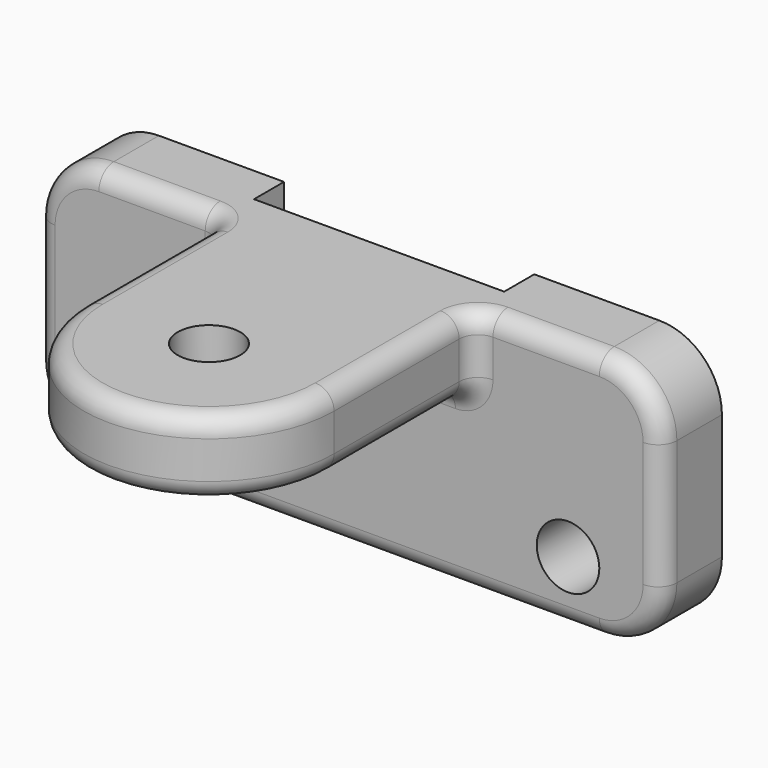
from build123d import *

# Parameters (mm, degrees)
F0_R      = 5
F1_DEPTH  = 12
F2_W      = 40
F2_H      = 40
F3_DEPTH  = 6
F4_W      = 40
F4_H      = 12
F5_DEPTH  = 28
F7_DEPTH  = 12
F8_F1_R   = 3
F8_F2_R   = 3
F9_R      = 3
F10_R     = 5
F11_DEPTH = 25


with BuildPart() as f1:
    # F0 (on Front) → F1 (new body)
    with BuildSketch(Plane.XZ):
        with BuildLine():
            Line((40, 20), (-40, 20))
            ThreePointArc((-40, 20), (-47.0710678119, 17.0710678119), (-50, 10))
            Line((-50, 10), (-50, -10))
            ThreePointArc((-50, -10), (-47.0710678119, -17.0710678119), (-40, -20))
            Line((-40, -20), (40, -20))
            ThreePointArc((40, -20), (47.0710678119, -17.0710678119), (50, -10))
            Line((50, -10), (50, 10))
            ThreePointArc((50, 10), (47.0710678119, 17.0710678119), (40, 20))
        make_face()
        with Locations((-35, -10)):
            Circle(F0_R, mode=Mode.SUBTRACT)
        with Locations((35, -10)):
            Circle(F0_R, mode=Mode.SUBTRACT)
    extrude(amount=F1_DEPTH)

    # F2 (on Front) → F3 (cut)
    with BuildSketch(Plane.XZ):
        Rectangle(F2_W, F2_H)
    extrude(amount=F3_DEPTH, mode=Mode.SUBTRACT)

    # F4 (on face) → F5 (join)
    with BuildSketch(Plane.XZ.offset(12)):
        with Locations((0, 14)):
            Rectangle(F4_W, F4_H)
    extrude(amount=F5_DEPTH)

    # F6 (on face) → F7 (join)
    with BuildSketch(Plane.XY.offset(20)):
        with BuildLine():
            Line((20, -40), (-20, -40))
            ThreePointArc((-20, -40), (0, -60), (20, -40))
        make_face()
    extrude(amount=-F7_DEPTH)

    # F8: fillet of radius 3 on 4 edges, made by hand

    # F8_f1
    f8_f1_edges = [f1.edges().sort_by_distance(p)[0] for p in [
        (-20, -26, 8),
        (0, -60, 8),
        (20, -26, 8),
    ]]
    fillet(f8_f1_edges, radius=F8_F1_R)

    # F8_f2
    f8_f2_edges = [f1.edges().sort_by_distance(p)[0] for p in [
        (0, -12, 8),
        (-19.1213203436, -12, 8.8786796564),
        (19.1213203436, -12, 8.8786796564),
    ]]
    fillet(f8_f2_edges, radius=F8_F2_R)

    # F9
    f9_edges = [f1.edges().sort_by_distance(p)[0] for p in [
        (-20, -40, 15.5),
        (0, -60, 11),
        (0, -60, 20),
        (20, -40, 15.5),
        (-31.5, -12, 20),
        (-47.071068, -12, 17.071068),
        (-50, -12, 0),
        (-47.071068, -12, -17.071068),
        (0, -12, -20),
        (47.071068, -12, -17.071068),
        (31.5, -12, 20),
        (50, -12, 0),
        (47.071068, -12, 17.071068),
        (20.87868, -12.87868, 20),
        (20, -27.5, 20),
        (-20, -27.5, 20),
        (-20.87868, -12.87868, 20),
    ]]
    fillet(f9_edges, radius=F9_R)

    # F10 (on face) → F11 (cut)
    with BuildSketch(Plane(origin=(0, 0, 8), x_dir=(1, 0, 0), z_dir=(0, 0, -1))):
        with Locations((0, 40)):
            Circle(F10_R)
    extrude(amount=-F11_DEPTH, mode=Mode.SUBTRACT)


solid = f1.part
